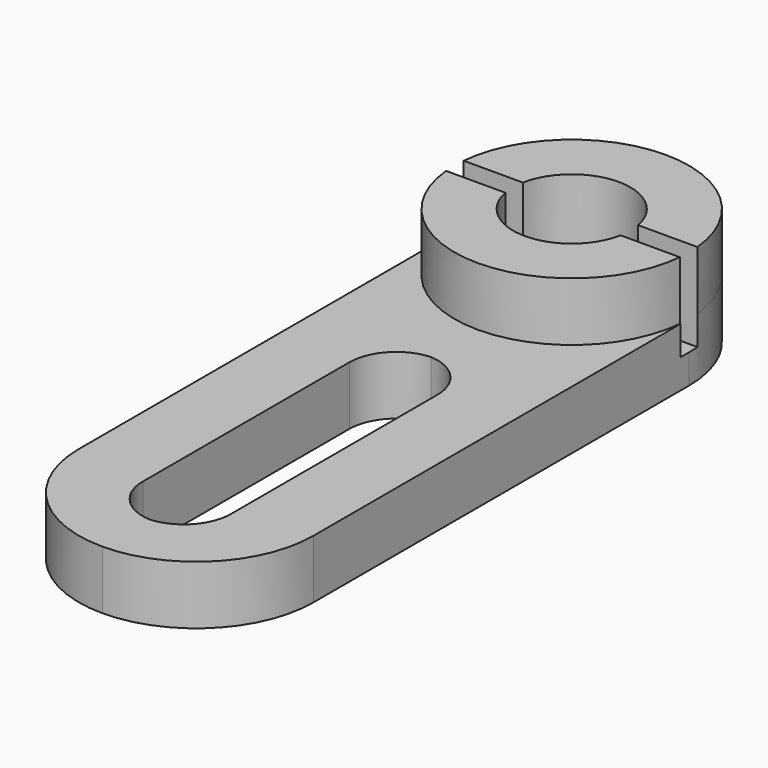
from build123d import *

# Parameters (mm, degrees)
F4_W         = 25.4
F4_H         = 76.2
F5_DEPTH     = 6.35
F6_R         = 12.7
F7_DEPTH     = 6.35
F8_R         = 6.35
F9_DEPTH     = 12.701
F10_W        = 25.4
F10_H        = 2.38125
F11_DEPTH    = 9.525
F12_W        = 9.525
F12_H        = 38.1
F13_DEPTH    = 6.351
F14_R        = 12.6999
F15_T1_DEPTH = 6.35


# Not quite as in the source:
# - a variable given as a bare number and used for a length is read in inches; the dataset says mm whatever the document's units were
# - a fillet or chamfer that OpenCascade refuses, or shapes differently, is made with other operations: its cross-section is extruded or revolved along the edge and cut away or added
# - a fillet or chamfer is up to 0.001 mm smaller than in the source, because OpenCascade refuses the exact size


with BuildPart() as f5:
    # F4 (on Top) → F5 (new body)
    with BuildSketch(Plane.XY):
        with Locations((12.7, 38.1)):
            Rectangle(F4_W, F4_H)
    extrude(amount=F5_DEPTH)

    # F6 (on face) → F7 (join)
    with BuildSketch(Plane.XY.offset(6.35)):
        with Locations((12.7, 63.5)):
            Circle(F6_R)
    extrude(amount=F7_DEPTH)

    # F8 (on face) → F9 (cut, through all)
    with BuildSketch(Plane.XY.offset(12.7)):
        with Locations((12.7, 63.5)):
            Circle(F8_R)
    extrude(amount=-F9_DEPTH, mode=Mode.SUBTRACT)

    # F10 (on face) → F11 (cut)
    with BuildSketch(Plane.XY.offset(12.7)):
        with Locations((12.7, 63.5)):
            Rectangle(F10_W, F10_H)
    extrude(amount=-F11_DEPTH, mode=Mode.SUBTRACT)

    # F12 (on face) → F13 (cut, through all)
    with BuildSketch(Plane.XY.offset(6.35)):
        with Locations((12.7, 25.4)):
            Rectangle(F12_W, F12_H)
    extrude(amount=-F13_DEPTH, mode=Mode.SUBTRACT)

    # F14 (radius 12.7 in the source; OpenCascade refuses exactly that, so slightly less here)
    f14_edges = [f5.edges().sort_by_distance(p)[0] for p in [
        (25.4, 0, 3.175),
        (0, 0, 3.175),
        (25.4, 76.2, 3.175),
        (0, 76.2, 3.175),
    ]]
    fillet(f14_edges, radius=F14_R)

    # F15: fillet of radius 5.08 on 4 edges, made by hand

    # F15_s2 → F15_t1 (join)
    with BuildSketch(Plane.XY):
        with BuildLine():
            ThreePointArc((17.4625, 11.43), (15.9746024484, 7.8378975516), (12.3825, 6.35))
            Line((12.3825, 6.35), (17.4625, 6.35))
            Line((17.4625, 6.35), (17.4625, 11.43))
        make_face()
        with BuildLine():
            ThreePointArc((7.9375, 11.43), (9.4253975516, 7.8378975516), (13.0175, 6.35))
            Line((13.0175, 6.35), (7.9375, 6.35))
            Line((7.9375, 6.35), (7.9375, 11.43))
        make_face()
        with BuildLine():
            ThreePointArc((13.0175, 44.45), (9.4253975516, 42.9621024484), (7.9375, 39.37))
            Line((7.9375, 39.37), (7.9375, 44.45))
            Line((7.9375, 44.45), (13.0175, 44.45))
        make_face()
        with BuildLine():
            ThreePointArc((17.4625, 39.37), (15.9746024484, 42.9621024484), (12.3825, 44.45))
            Line((12.3825, 44.45), (17.4625, 44.45))
            Line((17.4625, 44.45), (17.4625, 39.37))
        make_face()
    extrude(amount=F15_T1_DEPTH)


solid = f5.part
